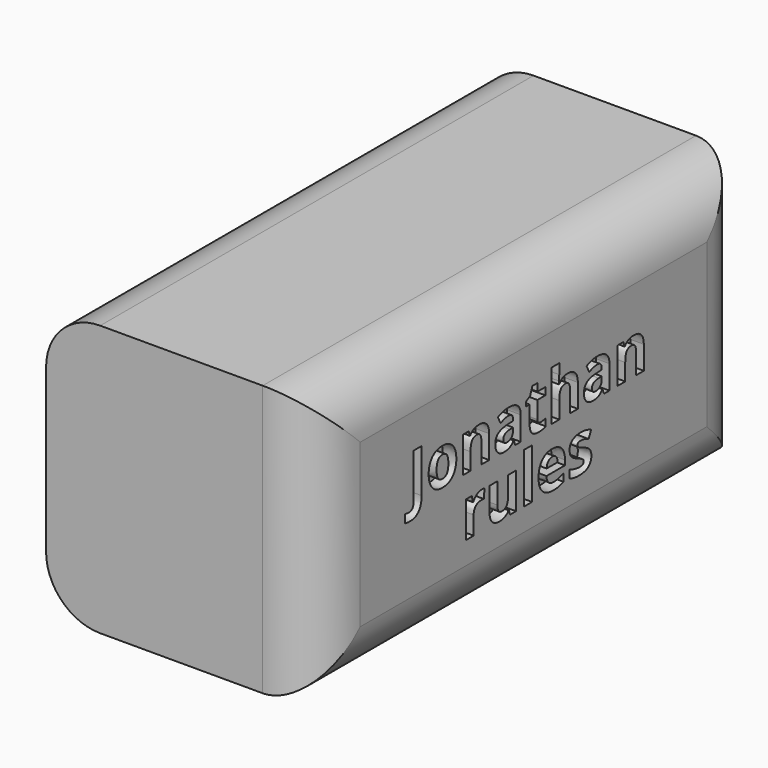
from build123d import *

# Parameters (mm, degrees)
F0_W           = 25.4
F0_H           = 25.4
F1_DEPTH       = 50.8
F3_R           = 5.08
F4_TEXT_SIZE   = 6.1336047818
F4_TEXT_SIZE_2 = 6.1629209085
F5_DEPTH       = 1.27


# Not quite as in the source:
# - a feature of the source that left no trace in its solid (it failed there, or was rolled back) is left out
# - Text() gives the source's letters only with a copy of the font that has no kerning and outlines rounded to 1/6400 em; it was checked with that copy


with BuildPart() as f1:
    # F0 (on Front) → F1 (new body)
    with BuildSketch(Plane.XZ):
        Rectangle(F0_W, F0_H)
    extrude(amount=F1_DEPTH)

    # F3
    f3_edges = [f1.edges().sort_by_distance(p)[0] for p in [
        (12.7, -50.8, 0),
        (12.7, 0, 0),
        (12.7, -25.4, -12.7),
        (12.7, -25.4, 12.7),
        (-12.7, -25.4, 12.7),
        (-12.7, -25.4, -12.7),
    ]]
    fillet(f3_edges, radius=F3_R)

    # F4 (on face) → F5 (cut)
    with BuildSketch(Plane.YZ.offset(12.7)):
        with Locations((-40.0021086452, 0)):
            Text('Jonathan', F4_TEXT_SIZE, font='Open Sans', font_style=FontStyle.BOLD, text_align=(TextAlign.LEFT, TextAlign.BOTTOM))
        with Locations((-33.8182151318, -5.5051520467)):
            Text('rules', F4_TEXT_SIZE_2, font='Open Sans', font_style=FontStyle.BOLD, text_align=(TextAlign.LEFT, TextAlign.BOTTOM))
    extrude(amount=-F5_DEPTH, mode=Mode.SUBTRACT)


solid = f1.part
